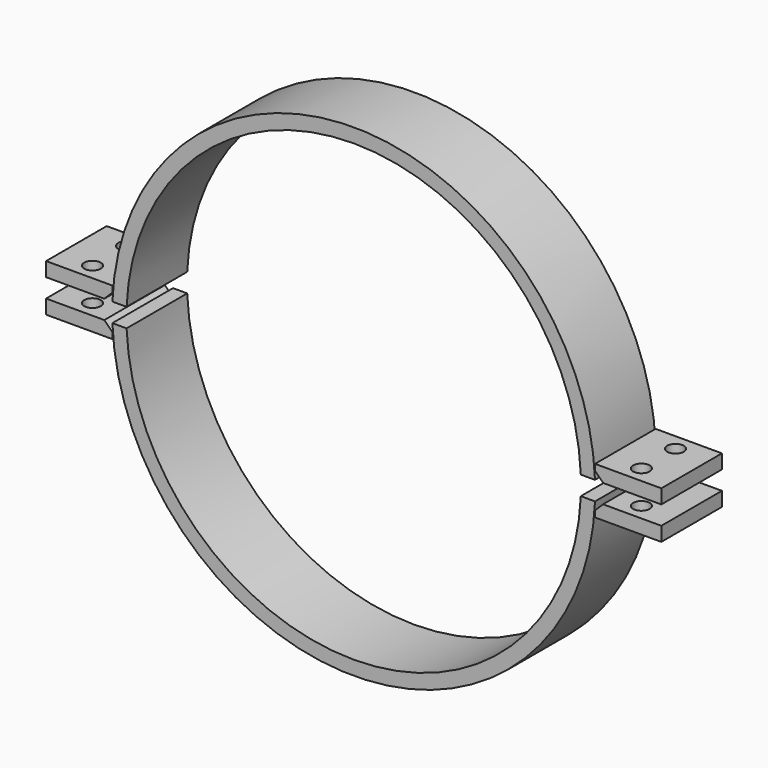
from build123d import *

# Parameters (mm, degrees)
F1_DEPTH = 101.6
F5_DEPTH = 101.6
F6_R     = 11.1125
F7_DEPTH = 25.4


# Not quite as in the source:
# - a feature of the source that left no trace in its solid (it failed there, or was rolled back) is left out


with BuildPart() as f1:
    # F0 (on Front) → F1 (new body)
    with BuildSketch(Plane.XZ):
        with BuildLine():
            ThreePointArc((-304.5353017304, 12.7), (0, 304.8), (304.5353017304, 12.7))
            Line((304.5353017304, 12.7), (323.6008845785, 12.7))
            ThreePointArc((323.6008845785, 12.7), (0, 323.85), (-323.6008845785, 12.7))
            Line((-323.6008845785, 12.7), (-304.5353017304, 12.7))
        make_face()
    extrude(amount=F1_DEPTH)


with BuildPart() as f2_1:
    # F2: instance of F1
    add(f1.part.mirror(Plane.XY))


with BuildPart() as f5:
    # F3 (on Front) → F5 (new body)
    with BuildSketch(Plane.XZ):
        Polygon((323.6008845785, 31.6401058242), (323.6008845785, 23.3883168548), (334.3990956091, 12.5901058242), (412.5008845785, 12.5901058242), (412.5008845785, 31.6401058242), align=None)
    extrude(amount=F5_DEPTH)

    # F6 (on face) → F7 (cut)
    with BuildSketch(Plane.XY.offset(31.6401058242)):
        with Locations((368.0508845785, -22.225)):
            Circle(F6_R)
        with Locations((368.0508845785, -79.375)):
            Circle(F6_R)
    extrude(amount=-F7_DEPTH, mode=Mode.SUBTRACT)


with BuildPart() as f8_1:
    # F8: instance of F5
    add(f5.part.mirror(Plane.YZ))


with BuildPart() as f9_1:
    # F9: instance of F8_1
    add(f8_1.part.mirror(Plane.XY))


with BuildPart() as f9_2:
    # F9: instance of F5
    add(f5.part.mirror(Plane.XY))


solid = Compound([f1.part, f2_1.part, f5.part, f8_1.part, f9_1.part, f9_2.part])
